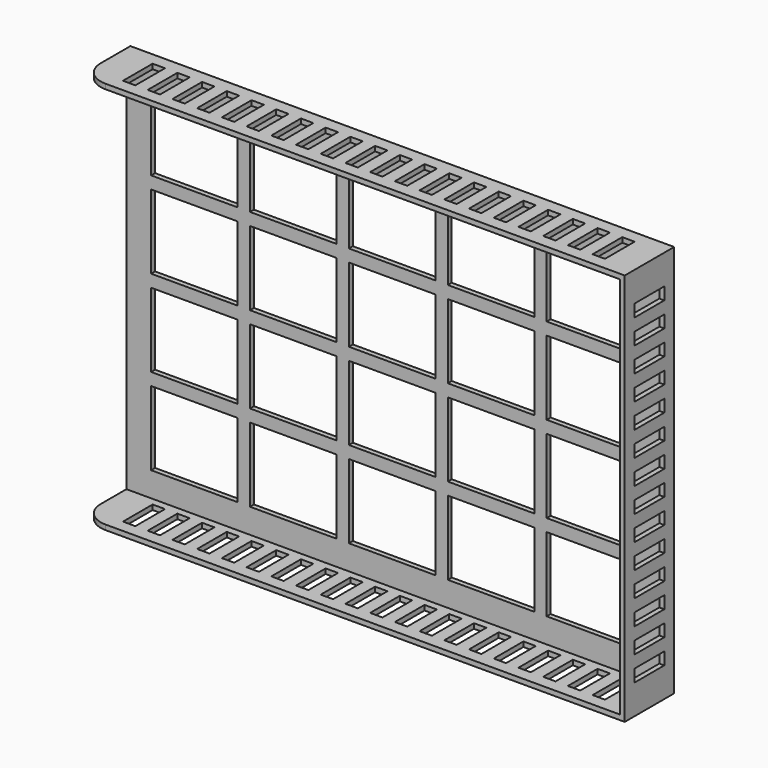
from build123d import *

# Parameters (mm, degrees)
F0_W      = 220
F0_H      = 159
F1_DEPTH  = 25
F2_T      = -2
F3_R      = 10
F5_W      = 35
F5_H      = 30
F6_DEPTH  = 25
F7_W      = 5
F7_H      = 15
F8_DEPTH  = 159.001
F9_W      = 15
F9_H      = 5
F10_DEPTH = 25


# Not quite as in the source:
# - two fillets or chamfers of one size are made in one step


with BuildPart() as f1:
    # F0 (on Front) → F1 (new body)
    with BuildSketch(Plane.XZ):
        Rectangle(F0_W, F0_H)
    extrude(amount=F1_DEPTH)

    # F2
    f2_openings = [f1.faces().sort_by_distance(p)[0] for p in [
        (0, -25, 0),
        (-110, -12.5, 0),
    ]]
    offset(amount=F2_T, openings=f2_openings)

    # F3
    f3_edges = [f1.edges().sort_by_distance(p)[0] for p in [
        (-110, -25, 78.5),
        (-110, -25, -78.5),
    ]]
    fillet(f3_edges, radius=F3_R)

    # F5 (on face) → F6 (cut)
    with BuildSketch(Plane.XZ.offset(2)):
        with Locations((-82.5, 52.5)):
            Rectangle(F5_W, F5_H)
        with Locations((-42.5, 52.5)):
            Rectangle(F5_W, F5_H)
        with Locations((-2.5, 52.5)):
            Rectangle(F5_W, F5_H)
        with Locations((37.5, 52.5)):
            Rectangle(F5_W, F5_H)
        with Locations((77.5, 52.5)):
            Rectangle(F5_W, F5_H)
        with Locations((77.5, 17.5)):
            Rectangle(F5_W, F5_H)
        with Locations((37.5, 17.5)):
            Rectangle(F5_W, F5_H)
        with Locations((-2.5, 17.5)):
            Rectangle(F5_W, F5_H)
        with Locations((-42.5, 17.5)):
            Rectangle(F5_W, F5_H)
        with Locations((-82.5, 17.5)):
            Rectangle(F5_W, F5_H)
        with Locations((-82.5, -17.5)):
            Rectangle(F5_W, F5_H)
        with Locations((-2.5, -17.5)):
            Rectangle(F5_W, F5_H)
        with Locations((37.5, -17.5)):
            Rectangle(F5_W, F5_H)
        with Locations((77.5, -17.5)):
            Rectangle(F5_W, F5_H)
        with Locations((77.5, -52.5)):
            Rectangle(F5_W, F5_H)
        with Locations((37.5, -52.5)):
            Rectangle(F5_W, F5_H)
        with Locations((-42.5, -52.5)):
            Rectangle(F5_W, F5_H)
        with Locations((-82.5, -52.5)):
            Rectangle(F5_W, F5_H)
        with Locations((-42.5, -17.5)):
            Rectangle(F5_W, F5_H)
        with Locations((-2.5, -52.5)):
            Rectangle(F5_W, F5_H)
    extrude(amount=-F6_DEPTH, mode=Mode.SUBTRACT)

    # F7 (on face) → F8 (cut, through all)
    with BuildSketch(Plane.XY.offset(79.5)):
        with Locations((95.5, -12.5)):
            Rectangle(F7_W, F7_H)
        with Locations((85.5, -12.5)):
            Rectangle(F7_W, F7_H)
        with Locations((75.5, -12.5)):
            Rectangle(F7_W, F7_H)
        with Locations((65.5, -12.5)):
            Rectangle(F7_W, F7_H)
        with Locations((55.5, -12.5)):
            Rectangle(F7_W, F7_H)
        with Locations((45.5, -12.5)):
            Rectangle(F7_W, F7_H)
        with Locations((35.5, -12.5)):
            Rectangle(F7_W, F7_H)
        with Locations((25.5, -12.5)):
            Rectangle(F7_W, F7_H)
        with Locations((15.5, -12.5)):
            Rectangle(F7_W, F7_H)
        with Locations((5.5, -12.5)):
            Rectangle(F7_W, F7_H)
        with Locations((-4.5, -12.5)):
            Rectangle(F7_W, F7_H)
        with Locations((-24.5, -12.5)):
            Rectangle(F7_W, F7_H)
        with Locations((-34.5, -12.5)):
            Rectangle(F7_W, F7_H)
        with Locations((-44.5, -12.5)):
            Rectangle(F7_W, F7_H)
        with Locations((-54.5, -12.5)):
            Rectangle(F7_W, F7_H)
        with Locations((-64.5, -12.5)):
            Rectangle(F7_W, F7_H)
        with Locations((-74.5, -12.5)):
            Rectangle(F7_W, F7_H)
        with Locations((-84.5, -12.5)):
            Rectangle(F7_W, F7_H)
        with Locations((-94.5, -12.5)):
            Rectangle(F7_W, F7_H)
        with Locations((-14.5, -12.5)):
            Rectangle(F7_W, F7_H)
    extrude(amount=-F8_DEPTH, mode=Mode.SUBTRACT)

    # F9 (on face) → F10 (cut)
    with BuildSketch(Plane.YZ.offset(110)):
        with Locations((-12.5, 65)):
            Rectangle(F9_W, F9_H)
        with Locations((-12.5, 55)):
            Rectangle(F9_W, F9_H)
        with Locations((-12.5, 45)):
            Rectangle(F9_W, F9_H)
        with Locations((-12.5, 35)):
            Rectangle(F9_W, F9_H)
        with Locations((-12.5, 25)):
            Rectangle(F9_W, F9_H)
        with Locations((-12.5, 15)):
            Rectangle(F9_W, F9_H)
        with Locations((-12.5, 5)):
            Rectangle(F9_W, F9_H)
        with Locations((-12.5, -5)):
            Rectangle(F9_W, F9_H)
        with Locations((-12.5, -15)):
            Rectangle(F9_W, F9_H)
        with Locations((-12.5, -25)):
            Rectangle(F9_W, F9_H)
        with Locations((-12.5, -35)):
            Rectangle(F9_W, F9_H)
        with Locations((-12.5, -45)):
            Rectangle(F9_W, F9_H)
        with Locations((-12.5, -55)):
            Rectangle(F9_W, F9_H)
        with Locations((-12.5, -65)):
            Rectangle(F9_W, F9_H)
    extrude(amount=-F10_DEPTH, mode=Mode.SUBTRACT)


solid = f1.part
